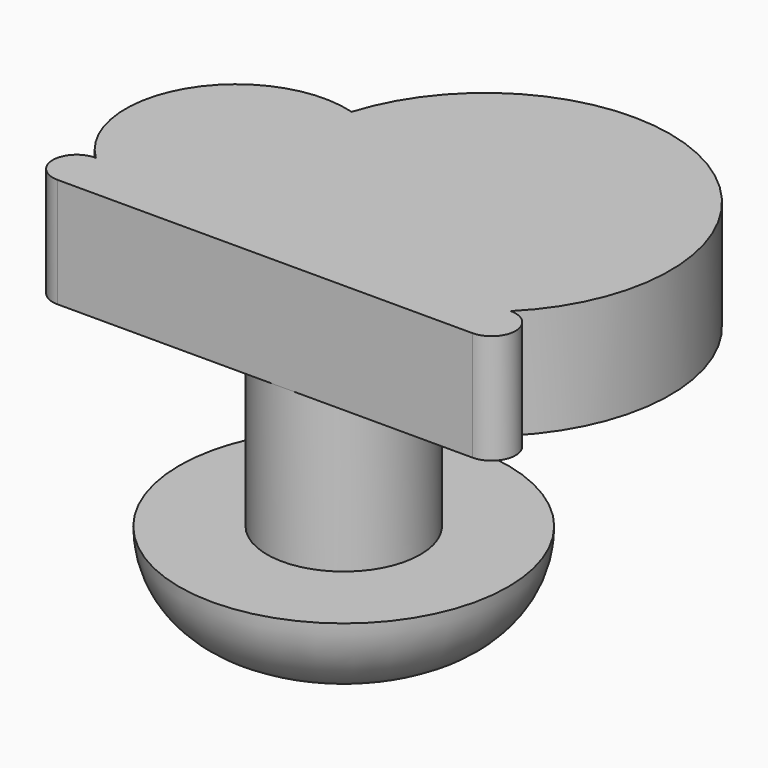
from build123d import *

# Parameters (mm, degrees)
F0_R     = 4.445
F1_DEPTH = 8.89
F3_DEPTH = 6.35
F4_R     = 9.525
F5_DEPTH = 5.08
F6_R     = 5.07999


# Not quite as in the source:
# - a fillet or chamfer is up to 0.001 mm smaller than in the source, because OpenCascade refuses the exact size


with BuildPart() as f1:
    # F0 (on Top) → F1 (new body)
    with BuildSketch(Plane.XY):
        Circle(F0_R)
    extrude(amount=F1_DEPTH)

    # F2 (on face) → F3 (join)
    with BuildSketch(Plane.XY.offset(8.89)):
        with BuildLine():
            Line((-13.0288261443, -4.445), (11.0172175353, -4.445))
            ThreePointArc((11.0172175353, -4.445), (12.4023835963, -3.0598339389), (11.0172175353, -1.6746678779))
            Line((11.0172175353, -1.6746678779), (-4.1174643288, -1.6746678779))
            Line((-4.1174643288, -1.6746678779), (-13.0288261443, -1.6746678779))
            ThreePointArc((-13.0288261443, -1.6746678779), (-14.4139922054, -3.0598339389), (-13.0288261443, -4.445))
        make_face()
        with BuildLine():
            Line((-4.1174643288, -1.6746678779), (11.0172175353, -1.6746678779))
            ThreePointArc((11.0172175353, -1.6746678779), (8.99040904, 15.1069926007), (-6.8009194972, 9.0765677298))
            ThreePointArc((-6.8009194972, 9.0765677298), (-2.3607405432, 4.4743080446), (-4.1174643288, -1.6746678779))
        make_face()
        with BuildLine():
            ThreePointArc((-6.8009194972, 9.0765677298), (-14.1136776733, 6.1332066084), (-13.0288261443, -1.6746678779))
            Line((-13.0288261443, -1.6746678779), (-4.1174643288, -1.6746678779))
            ThreePointArc((-4.1174643288, -1.6746678779), (-6.9553513424, 3.3275159413), (-6.8009194972, 9.0765677298))
        make_face()
        with BuildLine():
            ThreePointArc((-6.8009194972, 9.0765677298), (-6.9553513424, 3.3275159413), (-4.1174643288, -1.6746678779))
            ThreePointArc((-4.1174643288, -1.6746678779), (-2.3607405432, 4.4743080446), (-6.8009194972, 9.0765677298))
        make_face()
    extrude(amount=F3_DEPTH)

    # F4 (on face) → F5 (join)
    with BuildSketch(Plane(origin=(0, 0, 0), x_dir=(1, 0, 0), z_dir=(0, 0, -1))):
        Circle(F4_R)
    extrude(amount=F5_DEPTH)

    # F6 (radius 5.08 in the source; OpenCascade refuses exactly that, so slightly less here)
    f6_edges = [f1.edges().sort_by_distance(p)[0] for p in [
        (-9.525, 0, -5.08),
    ]]
    fillet(f6_edges, radius=F6_R)


solid = f1.part
